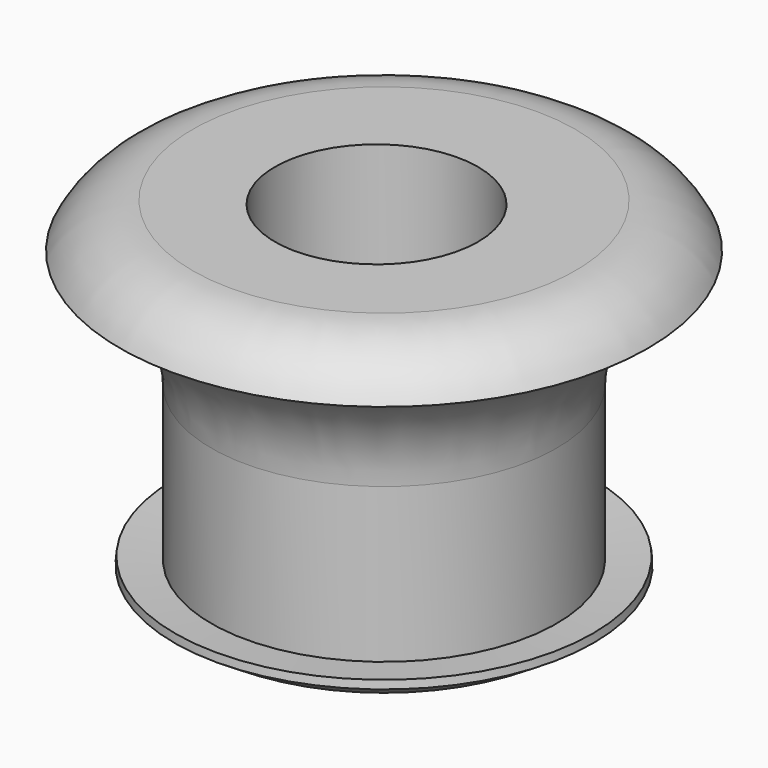
from build123d import *

# Parameters (mm, degrees)
F2_SIZE  = 0.3
F4_R     = 2.5
F5_DEPTH = 8


# Not quite as in the source:
# - a fillet or chamfer that OpenCascade refuses, or shapes differently, is made with other operations: its cross-section is extruded or revolved along the edge and cut away or added


with BuildPart() as f1:
    # F0 (on Right) → F1 (revolve)
    with BuildSketch(Plane.YZ):
        with BuildLine():
            Line((4.25, -6.8), (4.25, -3))
            ThreePointArc((4.25, -3), (4.878497412, -1.1651468819), (6.5, -0.1009926077))
            Line((6.5, -0.1009926077), (6.5, 1))
            Line((6.5, 1), (0, 1))
            Line((0, 1), (0, 0))
            Line((0, 0), (0, -7.5))
            Line((0, -7.5), (4.25, -7.5))
            Line((4.25, -7.5), (5.1640063768, -6.9207987711))
            Line((5.1640063768, -6.9207987711), (5.1465752283, -6.7215598315))
            Line((5.1465752283, -6.7215598315), (4.25, -6.8))
        make_face()
    revolve(axis=Axis((0, 0, -3.75), (0, 0, -1)))

    # F2
    f2_edges = [f1.edges().sort_by_distance(p)[0] for p in [
        (0, -4.25, -7.5),
    ]]
    chamfer(f2_edges, length=F2_SIZE)

    # F3: fillet of radius 2 on 1 edges, made by hand

    # F3_s1 → F3_t2 (revolve, cut)
    with BuildSketch(Plane.YZ):
        with BuildLine():
            ThreePointArc((6.5, -0.1009926077), (5.7627250062, 0.702647172), (4.7134430575, 1))
            Line((4.7134430575, 1), (6.5, 1))
            Line((6.5, 1), (6.5, -0.1009926077))
        make_face()
    revolve(axis=Axis((0, 0, 1), (0, 0, -1)), mode=Mode.SUBTRACT)

    # F4 (on face) → F5 (cut)
    with BuildSketch(Plane.XY.offset(1)):
        with Locations((0, -0.2312049229)):
            Circle(F4_R)
    extrude(amount=-F5_DEPTH, mode=Mode.SUBTRACT)


solid = f1.part
